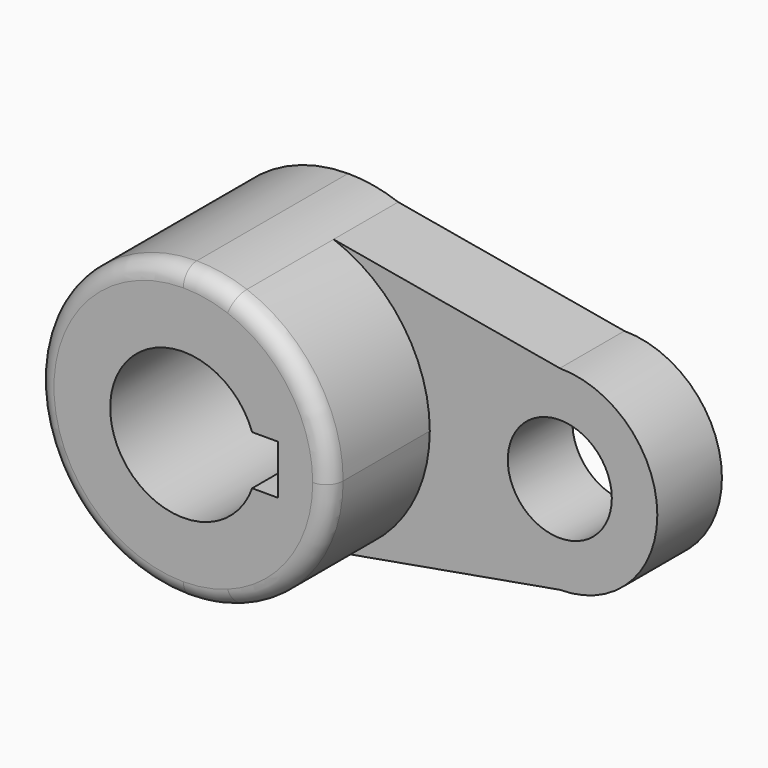
from build123d import *

# Parameters (mm, degrees)
F1_DEPTH = 40.2336
F0_R     = 10.16
F2_DEPTH = 15.7734
F3_R     = 3.302


with BuildPart() as f1:
    # F0 (on Front) → F1 (new body)
    with BuildSketch(Plane.XZ):
        with BuildLine():
            add(Edge.make_bspline(
                [(9.780704698, 26.8489932886), (6.5204697987, 27.4243288591), (3.2602348993, 27.9996644295), (0, 28.575)],
                knots=[44.8771660598, 44.8771660598, 44.8771660598, 44.8771660598, 54.8089978927, 54.8089978927, 54.8089978927, 54.8089978927], degree=3))
            ThreePointArc((0, 28.575), (-28.575, 0), (0, -28.575))
            add(Edge.make_bspline(
                [(9.780704698, -26.8489932886), (6.5204697987, -27.4243288591), (3.2602348993, -27.9996644295), (0, -28.575)],
                knots=[44.8771660598, 44.8771660598, 44.8771660598, 44.8771660598, 54.8089978927, 54.8089978927, 54.8089978927, 54.8089978927], degree=3))
            ThreePointArc((9.780704698, -26.8489932886), (23.4095521288, -16.3866864902), (28.575, 0))
            ThreePointArc((28.575, 0), (23.4095521288, 16.3866864902), (9.780704698, 26.8489932886))
        make_face()
        with BuildLine():
            ThreePointArc((13.4477648793, -4.826), (-14.2875, 0), (13.4477648793, 4.826))
            Line((13.4477648793, 4.826), (18.5293, 4.826))
            Line((18.5293, 4.826), (18.5293, -4.826))
            Line((18.5293, -4.826), (13.4477648793, -4.826))
        make_face(mode=Mode.SUBTRACT)
        with BuildLine():
            ThreePointArc((9.780704698, 26.8489932886), (4.9659159165, 28.1401901932), (0, 28.575))
            add(Edge.make_bspline(
                [(9.780704698, 26.8489932886), (6.5204697987, 27.4243288591), (3.2602348993, 27.9996644295), (0, 28.575)],
                knots=[44.8771660598, 44.8771660598, 44.8771660598, 44.8771660598, 54.8089978927, 54.8089978927, 54.8089978927, 54.8089978927], degree=3))
        make_face()
        with BuildLine():
            add(Edge.make_bspline(
                [(9.780704698, -26.8489932886), (6.5204697987, -27.4243288591), (3.2602348993, -27.9996644295), (0, -28.575)],
                knots=[44.8771660598, 44.8771660598, 44.8771660598, 44.8771660598, 54.8089978927, 54.8089978927, 54.8089978927, 54.8089978927], degree=3))
            ThreePointArc((0, -28.575), (4.9659159165, -28.1401901932), (9.780704698, -26.8489932886))
        make_face()
    extrude(amount=F1_DEPTH)

    # F0 (on Front) → F2 (join)
    with BuildSketch(Plane.XZ):
        with BuildLine():
            add(Edge.make_bspline(
                [(9.780704698, 26.8489932886), (6.5204697987, 27.4243288591), (3.2602348993, 27.9996644295), (0, 28.575)],
                knots=[44.8771660598, 44.8771660598, 44.8771660598, 44.8771660598, 54.8089978927, 54.8089978927, 54.8089978927, 54.8089978927], degree=3))
            ThreePointArc((0, 28.575), (-28.575, 0), (0, -28.575))
            add(Edge.make_bspline(
                [(9.780704698, -26.8489932886), (6.5204697987, -27.4243288591), (3.2602348993, -27.9996644295), (0, -28.575)],
                knots=[44.8771660598, 44.8771660598, 44.8771660598, 44.8771660598, 54.8089978927, 54.8089978927, 54.8089978927, 54.8089978927], degree=3))
            ThreePointArc((9.780704698, -26.8489932886), (23.4095521288, -16.3866864902), (28.575, 0))
            ThreePointArc((28.575, 0), (23.4095521288, 16.3866864902), (9.780704698, 26.8489932886))
        make_face()
        with BuildLine():
            ThreePointArc((13.4477648793, -4.826), (-14.2875, 0), (13.4477648793, 4.826))
            Line((13.4477648793, 4.826), (18.5293, 4.826))
            Line((18.5293, 4.826), (18.5293, -4.826))
            Line((18.5293, -4.826), (13.4477648793, -4.826))
        make_face(mode=Mode.SUBTRACT)
        with BuildLine():
            ThreePointArc((9.780704698, 26.8489932886), (4.9659159165, 28.1401901932), (0, 28.575))
            add(Edge.make_bspline(
                [(9.780704698, 26.8489932886), (6.5204697987, 27.4243288591), (3.2602348993, 27.9996644295), (0, 28.575)],
                knots=[44.8771660598, 44.8771660598, 44.8771660598, 44.8771660598, 54.8089978927, 54.8089978927, 54.8089978927, 54.8089978927], degree=3))
        make_face()
        with BuildLine():
            add(Edge.make_bspline(
                [(9.780704698, -26.8489932886), (6.5204697987, -27.4243288591), (3.2602348993, -27.9996644295), (0, -28.575)],
                knots=[44.8771660598, 44.8771660598, 44.8771660598, 44.8771660598, 54.8089978927, 54.8089978927, 54.8089978927, 54.8089978927], degree=3))
            ThreePointArc((0, -28.575), (4.9659159165, -28.1401901932), (9.780704698, -26.8489932886))
        make_face()
        with BuildLine():
            add(Edge.make_bspline(
                [(53.975, 19.05), (39.2435682327, 21.6496644295), (24.5121364653, 24.2493288591), (9.780704698, 26.8489932886)],
                knots=[0, 0, 0, 0, 44.8771660598, 44.8771660598, 44.8771660598, 44.8771660598], degree=3))
            ThreePointArc((9.780704698, 26.8489932886), (23.4095521288, 16.3866864902), (28.575, 0))
            ThreePointArc((28.575, 0), (23.4095521288, -16.3866864902), (9.780704698, -26.8489932886))
            add(Edge.make_bspline(
                [(53.975, -19.05), (39.2435682327, -21.6496644295), (24.5121364653, -24.2493288591), (9.780704698, -26.8489932886)],
                knots=[0, 0, 0, 0, 44.8771660598, 44.8771660598, 44.8771660598, 44.8771660598], degree=3))
            ThreePointArc((53.975, -19.05), (73.025, 0), (53.975, 19.05))
        make_face()
        with Locations((53.975, 0)):
            Circle(F0_R, mode=Mode.SUBTRACT)
    extrude(amount=F2_DEPTH)

    # F3
    f3_edges = [f1.edges().sort_by_distance(p)[0] for p in [
        (0, -40.2336, 28.575),
    ]]
    fillet(f3_edges, radius=F3_R)


solid = f1.part
